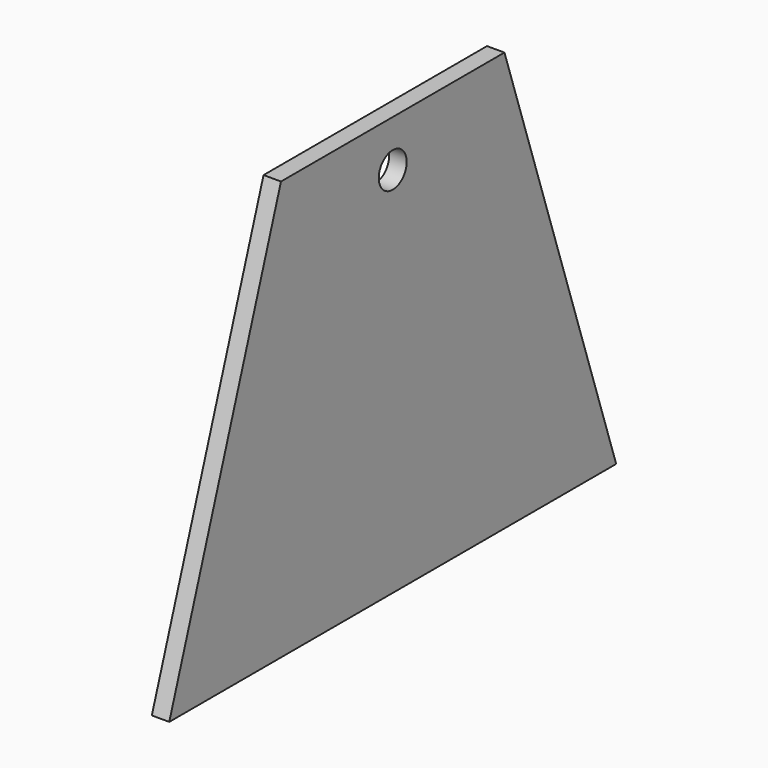
from build123d import *

# Parameters (mm, degrees)
F1_DEPTH = 19.05
F4_D     = 38.1


# Not quite as in the source:
# - the program builds the solid bodies; features that only make, move or delete a surface that nothing else refers to are left out


with BuildPart() as f1:
    # F0 (on Right) → F1 (new body)
    with BuildSketch(Plane.YZ):
        Polygon((-425.3114081136, -33.6309112608), (-272.9114081136, -33.6309112608), (31.8885918864, -33.6309112608), (184.2885918864, -33.6309112608), (31.8885918864, 423.5690887392), (-272.9114081136, 423.5690887392), align=None)
    extrude(amount=F1_DEPTH)

    # F4 (through all)
    with Locations(Plane(origin=(0, 0, 0), x_dir=(0, 1, 0), z_dir=(-1, 0, 0))):
        with Locations((-120.5114081136, -372.7690887392)):
            Hole(F4_D / 2)


solid = f1.part
